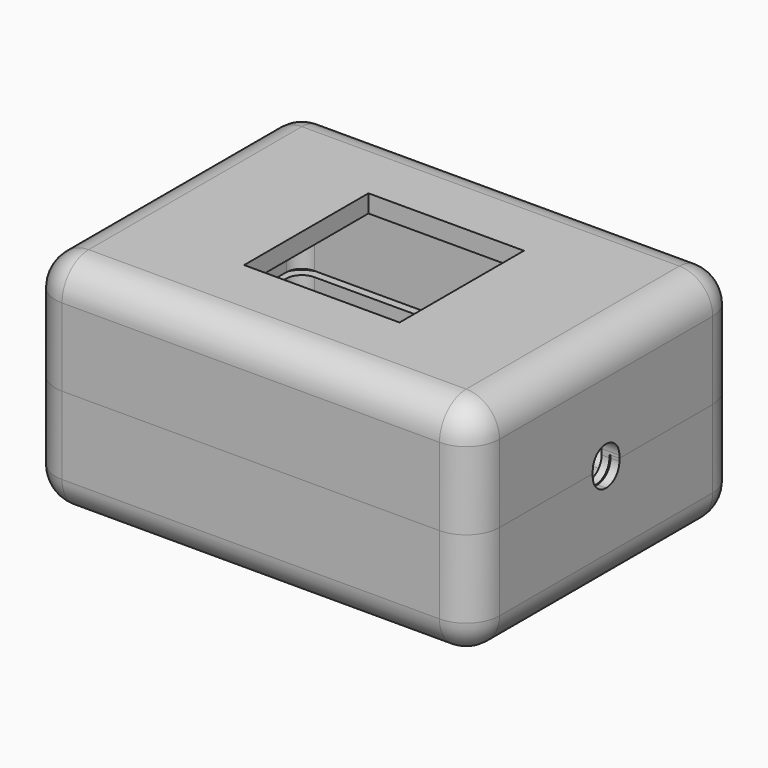
from build123d import *

# Parameters (mm, degrees)
F0_W      = 40
F0_H      = 30
F1_DEPTH  = 10
F2_DEPTH  = 10
F3_R      = 3
F3_2_R    = 3
F4_T      = -1.6
F5_T      = -1.6
F6_W      = 14
F6_H      = 14
F7_DEPTH  = 3
F9_DEPTH  = 2.5
F11_DEPTH = 2
F12_W     = 4
F12_H     = 1.5
F13_DEPTH = 5
F14_R     = 0.5
F14_2_R   = 0.5
F15_W     = 3
F15_H     = 1.75
F16_DEPTH = 5
F17_R     = 1.49999
F17_2_R   = 1.49999


# Not quite as in the source:
# - a fillet or chamfer is up to 0.001 mm smaller than in the source, because OpenCascade refuses the exact size
# - a feature names something its author has since deleted; it is built from what else it names


with BuildPart() as f1:
    # F0 (on Top) → F1 (new body)
    with BuildSketch(Plane.XY):
        with Locations((0.5547776818, 4.3791863923)):
            Rectangle(F0_W, F0_H)
    extrude(amount=F1_DEPTH)


with BuildPart() as f2:
    # F2 (new): a face of the model
    f2_faces = [f1.part.faces().sort_by_distance(p)[0] for p in [
        (0.5547776818, 4.3791863923, 0),
    ]]
    extrude(f2_faces, amount=F2_DEPTH)

    # F3
    f3_edges = [f2.edges().sort_by_distance(p)[0] for p in [
        (-19.445222, -10.620814, -5),
        (20.554778, -10.620814, -5),
        (20.554778, 19.379186, -5),
        (-19.445222, 19.379186, -5),
        (0.554778, 19.379186, -10),
        (-19.445222, 4.379186, -10),
        (0.554778, -10.620814, -10),
        (20.554778, 4.379186, -10),
    ]]
    fillet(f3_edges, radius=F3_R)

    # F4
    f4_openings = [f2.faces().sort_by_distance(p)[0] for p in [
        (0.554778, 4.379186, 0),
    ]]
    offset(amount=F4_T, openings=f4_openings)

    # F8 (on face) → F9 (cut)
    with BuildSketch(Plane.XY):
        with BuildLine():
            Line((19.7547776818, -7.6208136077), (19.7547776818, 16.3791863923))
            ThreePointArc((19.7547776818, 16.3791863923), (19.1104126004, 17.9348213109), (17.5547776818, 18.5791863923))
            Line((17.5547776818, 18.5791863923), (-16.4452223182, 18.5791863923))
            ThreePointArc((-16.4452223182, 18.5791863923), (-18.0008572368, 17.9348213109), (-18.6452223182, 16.3791863923))
            Line((-18.6452223182, 16.3791863923), (-18.6452223182, -7.6208136077))
            ThreePointArc((-18.6452223182, -7.6208136077), (-18.0008572368, -9.1764485263), (-16.4452223182, -9.8208136077))
            Line((-16.4452223182, -9.8208136077), (17.5547776818, -9.8208136077))
            ThreePointArc((17.5547776818, -9.8208136077), (19.1104126004, -9.1764485263), (19.7547776818, -7.6208136077))
        make_face()
        with BuildLine():
            ThreePointArc((17.5547776818, 17.7791863923), (18.5447271755, 17.369135886), (18.9547776818, 16.3791863923))
            Line((18.9547776818, 16.3791863923), (18.9547776818, -7.6208136077))
            ThreePointArc((18.9547776818, -7.6208136077), (18.5447271755, -8.6107631014), (17.5547776818, -9.0208136077))
            Line((17.5547776818, -9.0208136077), (-16.4452223182, -9.0208136077))
            ThreePointArc((-16.4452223182, -9.0208136077), (-17.4351718118, -8.6107631014), (-17.8452223182, -7.6208136077))
            Line((-17.8452223182, -7.6208136077), (-17.8452223182, 16.3791863923))
            ThreePointArc((-17.8452223182, 16.3791863923), (-17.4351718118, 17.369135886), (-16.4452223182, 17.7791863923))
            Line((-16.4452223182, 17.7791863923), (17.5547776818, 17.7791863923))
        make_face(mode=Mode.SUBTRACT)
    extrude(amount=-F9_DEPTH, mode=Mode.SUBTRACT)


with BuildPart() as f1_1:
    add(f1.part)

    # F3#2
    f3_2_edges = [f1_1.edges().sort_by_distance(p)[0] for p in [
        (-19.445222, -10.620814, 5),
        (20.554778, -10.620814, 5),
        (20.554778, 19.379186, 5),
        (-19.445222, 19.379186, 5),
        (20.554778, 4.379186, 10),
        (0.554778, 19.379186, 10),
        (-19.445222, 4.379186, 10),
        (0.554778, -10.620814, 10),
    ]]
    fillet(f3_2_edges, radius=F3_2_R)

    # F5
    f5_openings = [f1_1.faces().sort_by_distance(p)[0] for p in [
        (0.554778, 4.379186, 0),
    ]]
    offset(amount=F5_T, openings=f5_openings)

    # F6 (on face) → F7 (cut)
    with BuildSketch(Plane.XY.offset(10)):
        with Locations((0.5547776818, 4.3791863923)):
            Rectangle(F6_W, F6_H)
    extrude(amount=-F7_DEPTH, mode=Mode.SUBTRACT)

    # F10 (on face) → F11 (join)
    with BuildSketch(Plane(origin=(0, 0, 0), x_dir=(1, 0, 0), z_dir=(0, 0, -1))):
        with BuildLine():
            Line((19.6547776818, -16.3791863923), (19.6547776818, 7.6208136077))
            ThreePointArc((19.6547776818, 7.6208136077), (19.0397019223, 9.1057378482), (17.5547776818, 9.7208136077))
            Line((17.5547776818, 9.7208136077), (-16.4452223182, 9.7208136077))
            ThreePointArc((-16.4452223182, 9.7208136077), (-17.9301465587, 9.1057378482), (-18.5452223182, 7.6208136077))
            Line((-18.5452223182, 7.6208136077), (-18.5452223182, -16.3791863923))
            ThreePointArc((-18.5452223182, -16.3791863923), (-17.9301465587, -17.8641106328), (-16.4452223182, -18.4791863923))
            Line((-16.4452223182, -18.4791863923), (17.5547776818, -18.4791863923))
            ThreePointArc((17.5547776818, -18.4791863923), (19.0397019223, -17.8641106328), (19.6547776818, -16.3791863923))
        make_face()
        with BuildLine():
            ThreePointArc((17.5547776818, 9.0208136077), (18.5447271755, 8.6107631014), (18.9547776818, 7.6208136077))
            Line((18.9547776818, 7.6208136077), (18.9547776818, -16.3791863923))
            ThreePointArc((18.9547776818, -16.3791863923), (18.5447271755, -17.369135886), (17.5547776818, -17.7791863923))
            Line((17.5547776818, -17.7791863923), (-16.4452223182, -17.7791863923))
            ThreePointArc((-16.4452223182, -17.7791863923), (-17.4351718118, -17.369135886), (-17.8452223182, -16.3791863923))
            Line((-17.8452223182, -16.3791863923), (-17.8452223182, 7.6208136077))
            ThreePointArc((-17.8452223182, 7.6208136077), (-17.4351718118, 8.6107631014), (-16.4452223182, 9.0208136077))
            Line((-16.4452223182, 9.0208136077), (17.5547776818, 9.0208136077))
        make_face(mode=Mode.SUBTRACT)
    extrude(amount=F11_DEPTH)


with BuildPart() as f13_tool:
    # F12 (on face) → F13 (new body)
    with BuildSketch(Plane(origin=(-19.4452223182, 0, 0), x_dir=(0, -1, 0), z_dir=(-1, 0, 0))):
        with Locations((-4.3791863923, -0.75)):
            Rectangle(F12_W, F12_H)
        with Locations((-4.3791863923, 0.75)):
            Rectangle(F12_W, F12_H)
    extrude(amount=-F13_DEPTH)


with BuildPart() as f1_2:
    add(f1_1.part)

    # F13: cut by f13_tool
    add(f13_tool.part, mode=Mode.SUBTRACT)

    # F14#2
    f14_2_edges = [f1_2.edges().sort_by_distance(p)[0] for p in [
        (-18.195222, 6.379186, -1.5),
        (-18.195222, 2.379186, -1.5),
        (-18.645222, 6.379186, 1.5),
        (-18.645222, 2.379186, 1.5),
    ]]
    fillet(f14_2_edges, radius=F14_2_R)


with BuildPart() as f2_1:
    add(f2.part)

    # F13: cut by f13_tool
    add(f13_tool.part, mode=Mode.SUBTRACT)

    # F14
    f14_edges = [f2_1.edges().sort_by_distance(p)[0] for p in [
        (-19.045222, 6.379186, -1.5),
        (-19.045222, 2.379186, -1.5),
    ]]
    fillet(f14_edges, radius=F14_R)


with BuildPart() as f16_tool:
    # F15 (on face) → F16 (new body)
    with BuildSketch(Plane.YZ.offset(20.5547776818)):
        with Locations((4.3791863923, 0.875)):
            Rectangle(F15_W, F15_H)
        with Locations((4.3791863923, -0.875)):
            Rectangle(F15_W, F15_H)
    extrude(amount=-F16_DEPTH)


with BuildPart() as f1_3:
    add(f1_2.part)

    # F16: cut by f16_tool
    add(f16_tool.part, mode=Mode.SUBTRACT)

    # F17 (radius 1.5 in the source; OpenCascade refuses exactly that, so slightly less here)
    f17_edges = [f1_3.edges().sort_by_distance(p)[0] for p in [
        (19.304778, 2.879186, -1.75),
        (19.304778, 5.879186, -1.75),
        (19.754778, 2.879186, 1.75),
        (19.754778, 5.879186, 1.75),
    ]]
    fillet(f17_edges, radius=F17_R)


with BuildPart() as f2_2:
    add(f2_1.part)

    # F16: cut by f16_tool
    add(f16_tool.part, mode=Mode.SUBTRACT)

    # F17#2 (radius 1.5 in the source; OpenCascade refuses exactly that, so slightly less here)
    f17_2_edges = [f2_2.edges().sort_by_distance(p)[0] for p in [
        (20.154778, 2.879186, -1.75),
        (20.154778, 5.879186, -1.75),
    ]]
    fillet(f17_2_edges, radius=F17_2_R)


solid = Compound([f1_3.part, f2_2.part])
